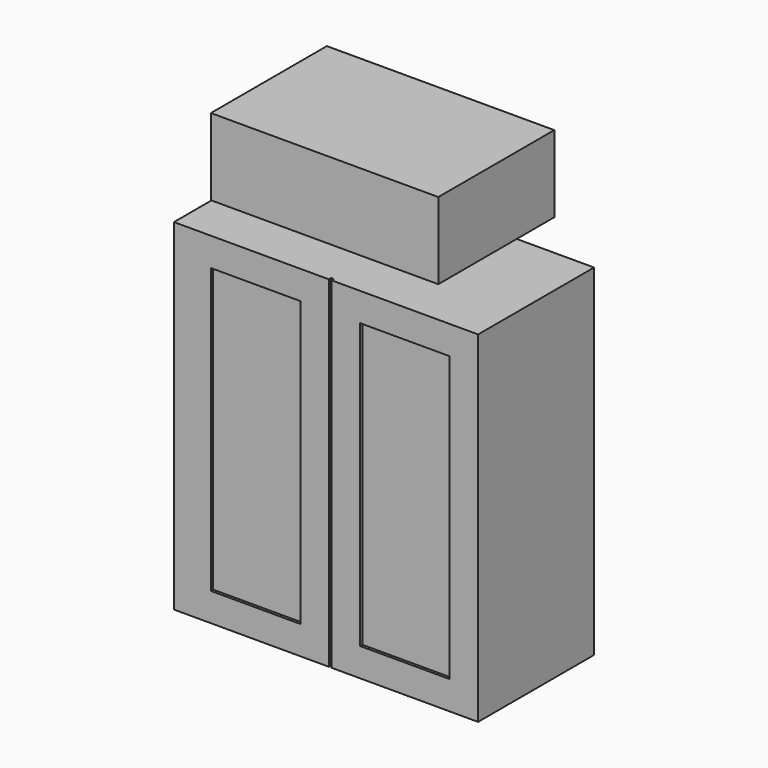
from build123d import *

# Parameters (mm, degrees)
F0_W     = 508
F0_H     = 171.45
F1_DEPTH = 323.85
F0_W_2   = 327.025
F0_H_2   = 762
F0_W_3   = 200.025
F0_H_3   = 635
F2_DEPTH = 6.35
F3_W     = 323.85
F3_H     = 762
F3_W_2   = 196.85
F3_H_2   = 635
F4_DEPTH = 19.05
F5_DEPTH = 12.7


# Not quite as in the source:
# - a feature names something its author has since deleted; it is built from what else it names


with BuildPart() as f1:
    # F0 (on Front) → F1 (new body)
    with BuildSketch(Plane.XZ):
        with Locations((317.5, 917.575)):
            Rectangle(F0_W, F0_H)
    extrude(amount=-F1_DEPTH)


with BuildPart() as f1b:
    # F0 (on Front) → F1, piece 2 (new body)
    with BuildSketch(Plane.XZ):
        with Locations((163.5125, 381)):
            Rectangle(F0_W_2, F0_H_2)
        with Locations((163.5125, 381)):
            Rectangle(F0_W_3, F0_H_3, mode=Mode.SUBTRACT)
        with Locations((496.8875, 381)):
            Rectangle(F0_W_2, F0_H_2)
        with Locations((496.8875, 381)):
            Rectangle(F0_W_3, F0_H_3, mode=Mode.SUBTRACT)
        with Locations((163.5125, 381)):
            Rectangle(F0_W_3, F0_H_3)
        with Locations((496.8875, 381)):
            Rectangle(F0_W_3, F0_H_3)
        Polygon((327.025, 762), (327.025, 0), (333.375, 0), (333.375, 762), (330.2, 762), align=None)
    extrude(amount=-F1_DEPTH)

    # F0 (on Front) → F2 (cut)
    with BuildSketch(Plane.XZ):
        Polygon((327.025, 762), (327.025, 0), (333.375, 0), (333.375, 762), (330.2, 762), align=None)
        with Locations((317.5, 917.575)):
            Rectangle(F0_W, F0_H)
        with Locations((496.8875, 381)):
            Rectangle(F0_W_3, F0_H_3)
        with Locations((163.5125, 381)):
            Rectangle(F0_W_3, F0_H_3)
    extrude(amount=-F2_DEPTH, mode=Mode.SUBTRACT)

    # F3 (on face) → F4 (join)
    with BuildSketch(Plane(origin=(0, 0, 0), x_dir=(0, -1, 0), z_dir=(-1, 0, 0))):
        with Locations((-161.925, 381)):
            Rectangle(F3_W, F3_H)
        with Locations((-161.925, 381)):
            Rectangle(F3_W_2, F3_H_2, mode=Mode.SUBTRACT)
    extrude(amount=F4_DEPTH)

    # F5 (add): a face of the model
    f5_faces = [f1b.faces().sort_by_distance(p)[0] for p in [
        (0, 161.925, 381),
    ]]
    extrude(f5_faces, amount=F5_DEPTH)


solid = Compound([f1.part, f1b.part])
